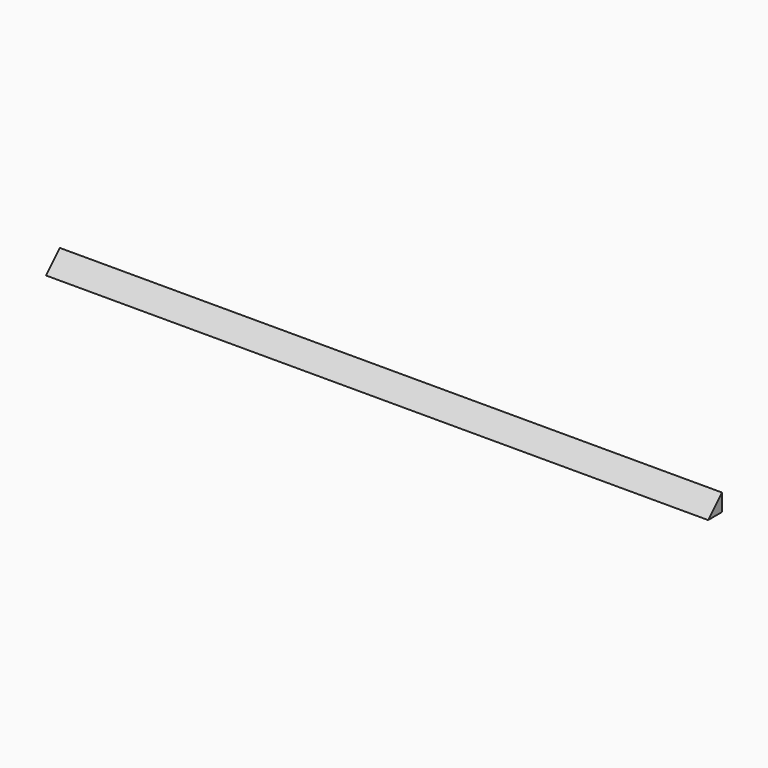
from build123d import *

# Parameters (mm, degrees)
F0_W        = 730.25
F0_H        = 25.4
F1_DEPTH    = 19.05
F2_T1_DEPTH = 860.8914957887


# Not quite as in the source:
# - a fillet or chamfer that OpenCascade refuses, or shapes differently, is made with other operations: its cross-section is extruded or revolved along the edge and cut away or added


with BuildPart() as f1:
    # F0 (on Front) → F1 (new body)
    with BuildSketch(Plane.XZ):
        Rectangle(F0_W, F0_H)
    extrude(amount=F1_DEPTH)

    # F2: chamfer of 25.4 on 1 edges, made by hand

    # F2_s2 → F2_t1 (cut)
    with BuildSketch(Plane.YZ.offset(-430.4457478943)):
        Polygon((6.35, 12.7), (-19.05, -12.7), (-19.05, 12.7), align=None)
    extrude(amount=F2_T1_DEPTH, mode=Mode.SUBTRACT)


solid = f1.part
